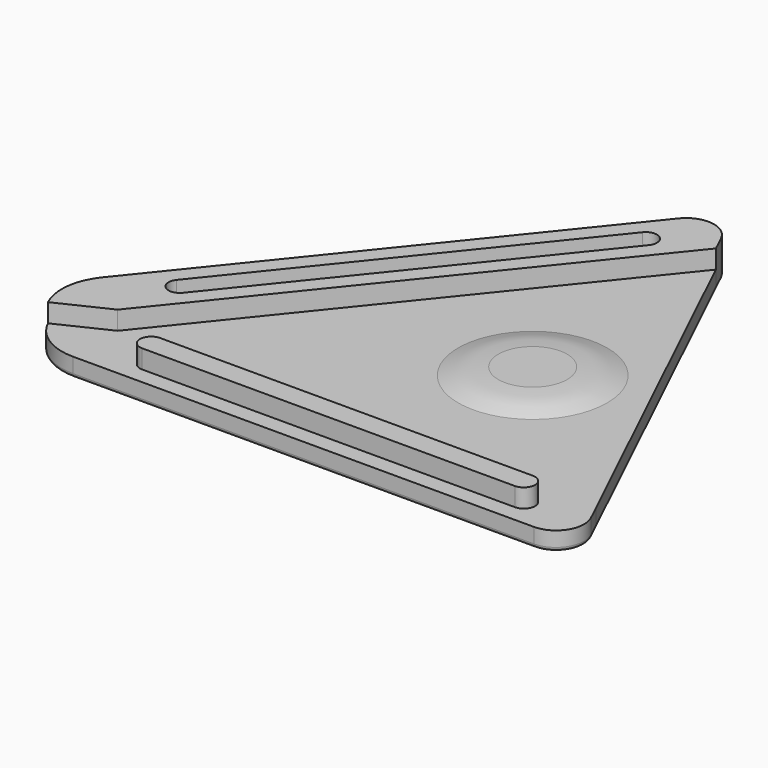
from build123d import *

# Parameters (mm, degrees)
F2_DEPTH    = 1
F4_DEPTH    = 1
F5_T1_DEPTH = 13.9032439889
F5_T3_DEPTH = 12.9032439889
F6_R        = 4
F7_DEPTH    = 0.4
F10_R       = 0.2


# Not quite as in the source:
# - a fillet or chamfer that OpenCascade refuses, or shapes differently, is made with other operations: its cross-section is extruded or revolved along the edge and cut away or added


with BuildPart() as f2:
    # F0 (on Top) → F2 (new body)
    with BuildSketch(Plane.XY):
        Polygon((0, 20), (-16.1091689951, 0), (9.5716667723, 0), align=None)
    extrude(amount=F2_DEPTH)



with BuildPart() as f2b:
    # F1 (on face) → F2, piece 2 (new body)
    with BuildSketch(Plane.XY):
        with BuildLine():
            Line((-1.4357500158, 23), (-18.4455415549, 1.8818510201))
            ThreePointArc((-18.4455415549, 1.8818510201), (-18.8152319157, -1.295076627), (-16.1091689951, -3))
            Line((-16.1091689951, -3), (11.0074167882, -3))
            Line((11.0074167882, -3), (9.5716667723, 0))
            Line((9.5716667723, 0), (-16.1091689951, 0))
            Line((-16.1091689951, 0), (0, 20))
            Line((0, 20), (-1.4357500158, 23))
        make_face()
    extrude(amount=F2_DEPTH)


with BuildPart() as f2_1:
    add(f2.part)

    add(f2b.part)  # F4 merges F2b
    # F3 (on face) → F4 (join)
    with BuildSketch(Plane.XY.offset(1)):
        with BuildLine():
            Line((-18.8152319157, -1.295076627), (-16.1091689951, 0))
            Line((-16.1091689951, 0), (0, 20))
            Line((0, 20), (-1.4357500158, 23))
            Line((-1.4357500158, 23), (-18.4455415549, 1.8818510201))
            ThreePointArc((-18.4455415549, 1.8818510201), (-19.0890609751, 0.3467618604), (-18.8152319157, -1.295076627))
        make_face()
        with BuildLine():
            ThreePointArc((-14.928229743, 2.9009278658), (-15.771874459, 2.8100235579), (-15.8627787669, 3.6536682739))
            Line((-15.8627787669, 3.6536682739), (-3.3171052997, 19.2294853393))
            ThreePointArc((-3.3171052997, 19.2294853393), (-2.4734605837, 19.3203896472), (-2.3825562758, 18.4767449312))
            Line((-2.3825562758, 18.4767449312), (-14.928229743, 2.9009278658))
        make_face(mode=Mode.SUBTRACT)
        with BuildLine():
            Line((6.8908310049, -0.9), (-13.1091689951, -0.9))
            ThreePointArc((-13.1091689951, -0.9), (-13.7091689951, -1.5), (-13.1091689951, -2.1))
            Line((-13.1091689951, -2.1), (6.8908310049, -2.1))
            ThreePointArc((6.8908310049, -2.1), (7.4908310049, -1.5), (6.8908310049, -0.9))
        make_face()
    extrude(amount=F4_DEPTH)

    # F5: fillet of radius 1.5 on 2 edges, made by hand

    # F5_s2 → F5_t1 (cut)
    with BuildSketch(Plane.XY.offset(-5.9516219944)):
        with BuildLine():
            ThreePointArc((-0.4079522763, 20.8526480249), (-1.5876028064, 21.6950557014), (-2.9291700165, 21.1460352214))
            Line((-2.9291700165, 21.1460352214), (-2.9525337421, 21.1648537316))
            ThreePointArc((-2.9525337421, 21.1648537316), (-2.2057848022, 22.0918047567), (-1.4591137414, 23.0188185102))
            Line((-1.4591137414, 23.0188185102), (-1.4086893866, 23.0129507663))
            ThreePointArc((-1.4086893866, 23.0129507663), (-0.8948356179, 21.9392531941), (-0.3808916471, 20.8655987912))
            Line((-0.3808916471, 20.8655987912), (-0.4079522763, 20.8526480249))
        make_face()
    extrude(amount=F5_T1_DEPTH, mode=Mode.SUBTRACT)

    # F5_s4 → F5_t3 (cut)
    with BuildSketch(Plane.XY.offset(-5.9516219944)):
        with BuildLine():
            ThreePointArc((9.9797994528, -0.8525616865), (9.8958833281, -2.2996913111), (8.6267679925, -3.0001))
            Line((8.6267679925, -3.0001), (8.6267679925, -3.0301))
            ThreePointArc((8.6267679925, -3.0301), (9.8170923903, -3.03), (11.0074167882, -3.03))
            Line((11.0074167882, -3.03), (11.0344774174, -2.9870492337))
            ThreePointArc((11.0344774174, -2.9870492337), (10.5206236486, -1.9133516616), (10.006860082, -0.8396109202))
            Line((10.006860082, -0.8396109202), (9.9797994528, -0.8525616865))
        make_face()
    extrude(amount=F5_T3_DEPTH, mode=Mode.SUBTRACT)

    # F6 (on face) → F7 (join)
    with BuildSketch(Plane.XY.offset(1)):
        with Locations((0, 7.70957988)):
            Circle(F6_R)
    extrude(amount=F7_DEPTH)

    # F8: fillet of radius 6 on 1 edges, made by hand

    # F8_s1 → F8_t2 (revolve, cut)
    with BuildSketch(Plane.XZ.offset(-7.70957988)):
        with BuildLine():
            ThreePointArc((4, 1), (2.9413791922, 1.2991524815), (1.8459340771, 1.4))
            Line((1.8459340771, 1.4), (4, 1.4))
            Line((4, 1.4), (4, 1))
        make_face()
    revolve(axis=Axis((0, 7.70957988, 1.4), (0, 0, 1)), mode=Mode.SUBTRACT)

    # F9: union 

    # F10
    f10_edges = [f2_1.edges().sort_by_distance(p)[0] for p in [
        (4.785833, 10, 0),
        (-1.587603, 21.695056, 0),
        (-10.681885, 11.520656, 0),
        (-18.815232, -1.295077, 0),
        (-3.73254, -3, 0),
        (9.895883, -2.299691, 0),
    ]]
    fillet(f10_edges, radius=F10_R)


solid = f2_1.part
